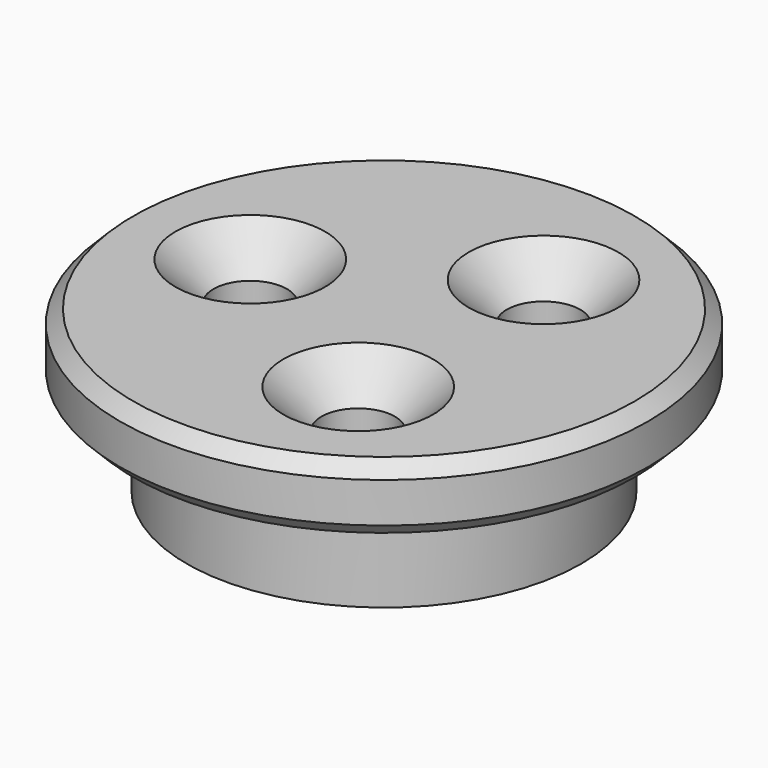
from build123d import *

# Parameters (mm, degrees)
F0_R            = 14.75
F2_DEPTH        = 7
F3_R            = 19.75
F3_R_2          = 14.75
F4_DEPTH        = 5
F6_D            = 5.5
F6_CSINK_D      = 11.2
F6_CSINK_ANGLE  = 90
F6_COPIES_COUNT = 3
F7_SIZE         = 1


# Not quite as in the source:
# - a pattern or mirror of a feature is missing from the dataset's text; its kind, count and spacing are read off the source's solid


with BuildPart() as f2:
    # F0 (on Top) → F2 (new body)
    with BuildSketch(Plane.XY):
        Circle(F0_R)
    extrude(amount=-F2_DEPTH)

    # F3 (on face) → F4 (join)
    with BuildSketch(Plane.XY):
        Circle(F3_R)
        Circle(F3_R_2, mode=Mode.SUBTRACT)
        Circle(F3_R_2)
    extrude(amount=F4_DEPTH)

    # F6 (through all)
    with Locations(Plane.XY.offset(5)):
        with Locations((-10, 0)):
            f6 = CounterSinkHole(F6_D / 2, F6_CSINK_D / 2, counter_sink_angle=F6_CSINK_ANGLE)

    # F6_copies: F6 ×3 about axis
    f6_copies_axis = Axis((0, 0, 0), (0, 0, 1))
    for i in range(1, F6_COPIES_COUNT):
        add(f6.rotate(f6_copies_axis, i * 360 / F6_COPIES_COUNT), mode=Mode.SUBTRACT)

    # F7
    f7_edges = [f2.edges().sort_by_distance(p)[0] for p in [
        (-19.75, 0, 5),
        (-19.75, 0, 0),
    ]]
    chamfer(f7_edges, length=F7_SIZE)


solid = f2.part
